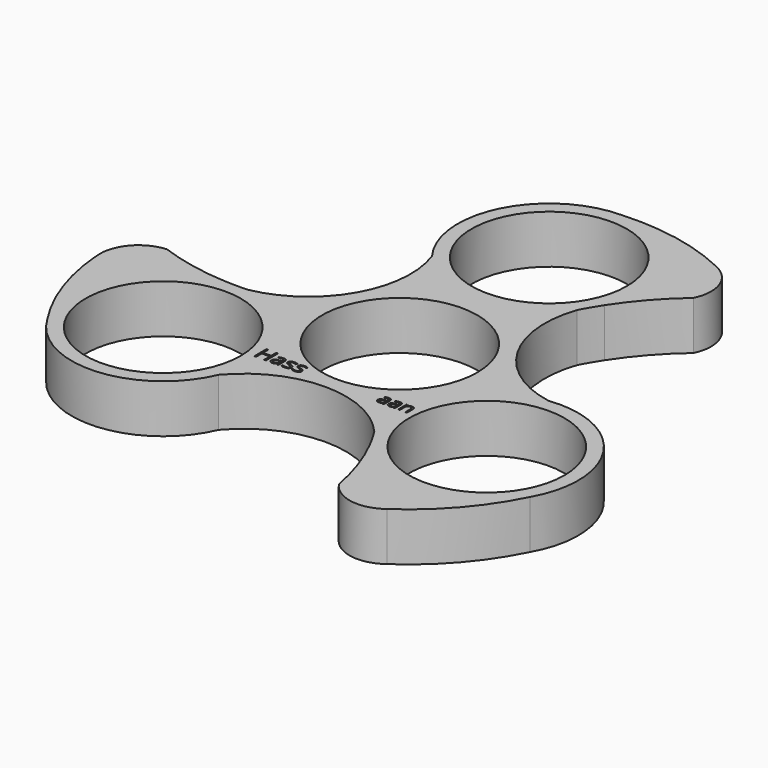
from build123d import *

# Parameters (mm, degrees)
F0_R         = 11.2
F1_DEPTH     = 7
F2_TEXT_SIZE = 3.0873436845
F3_DEPTH     = 13.4
F4_TEXT_SIZE = 2.8406800185
F5_DEPTH     = 9.9
F8_DEPTH     = 25


# Not quite as in the source:
# - Text() gives the source's letters only with a copy of the font that has no kerning and outlines rounded to 1/6400 em; it was checked with that copy


with BuildPart() as f1:
    # F0 (on Top) → F1 (new body)
    with BuildSketch(Plane.XY):
        with BuildLine():
            ThreePointArc((21.7602352684, -0.3790794713), (11.6629101979, 6.6669216362), (10.4657940357, 18.9212685418))
            ThreePointArc((10.4657940357, 18.9212685418), (11.2692033032, 20.371870284), (12.1401373601, 21.7829640918))
            ThreePointArc((12.1401373601, 21.7829640918), (17.0059122311, 27.7261145683), (23.0465047061, 32.4703790247))
            ThreePointArc((23.0465047061, 32.4703790247), (12.2370493927, 38.5690257647), (-0.0710858988, 40.165152914))
            ThreePointArc((-0.0710858988, 40.165152914), (-11.8253179711, 32.8306537694), (-10.551825182, 19.0344562705))
            ThreePointArc((-10.551825182, 19.0344562705), (-11.605178601, 6.7669156953), (-21.6191962469, -0.3969907652))
            ThreePointArc((-21.6191962469, -0.3969907652), (-23.2771588402, -0.426518801), (-24.9346689532, -0.3778146866))
            ThreePointArc((-24.9346689532, -0.3778146866), (-32.5144756799, 0.8644947226), (-39.643425459, 3.7236690316))
            ThreePointArc((-39.643425459, 3.7236690316), (-39.5202808078, -8.6869172409), (-34.748499821, -20.1441386512))
            ThreePointArc((-34.748499821, -20.1441386512), (-22.5195212016, -26.6563526555), (-11.2084100865, -18.6553767991))
            ThreePointArc((-11.2084100865, -18.6553767991), (-0.0577315969, -13.4338373316), (11.1534022111, -18.5242777766))
            ThreePointArc((11.1534022111, -18.5242777766), (12.0079555369, -19.945351483), (12.7945315932, -21.4051494051))
            ThreePointArc((12.7945315932, -21.4051494051), (15.5085634488, -28.5906092908), (16.5969207529, -36.1940480563))
            ThreePointArc((16.5969207529, -36.1940480563), (27.2832314151, -29.8821085238), (34.8195857199, -20.0210142628))
            ThreePointArc((34.8195857199, -20.0210142628), (34.3448391727, -6.1743011139), (21.7602352684, -0.3790794713))
        make_face()
        with Locations((-23.352673207, -13.4826721624)):
            Circle(F0_R, mode=Mode.SUBTRACT)
        Circle(F0_R, mode=Mode.SUBTRACT)
        with Locations((23.352673207, -13.4826721624)):
            Circle(F0_R, mode=Mode.SUBTRACT)
        with Locations((0, 26.9653443247)):
            Circle(F0_R, mode=Mode.SUBTRACT)
    extrude(amount=F1_DEPTH)

    # F2 (on face) → F3 (cut)
    with BuildSketch(Plane.XY.offset(7)):
        with Locations((-11.2112455724, -12.6004500012)):
            Text('Hass', F2_TEXT_SIZE, font='Open Sans', text_align=(TextAlign.LEFT, TextAlign.BOTTOM))
    extrude(amount=-F3_DEPTH, mode=Mode.SUBTRACT)

    # F4 (on face) → F5 (cut)
    with BuildSketch(Plane.XY.offset(7)):
        with Locations((6.4620403573, -12.6233948395)):
            Text('aan', F4_TEXT_SIZE, font='Open Sans', text_align=(TextAlign.LEFT, TextAlign.BOTTOM))
    extrude(amount=-F5_DEPTH, mode=Mode.SUBTRACT)

    # F7 (on face) → F8 (cut)
    with BuildSketch(Plane.XY.offset(7)):
        with BuildLine():
            ThreePointArc((-40.0765575469, -4.6404949389), (-38.8078254704, -0.355440868), (-34.801337868, 1.6243132995))
            ThreePointArc((-34.801337868, 1.6243132995), (-44.0770225904, 4.0814343372), (-40.0765575469, -4.6404949389))
        make_face()
        with BuildLine():
            ThreePointArc((24.0570652767, -32.3870694623), (19.7117335565, -33.430842289), (15.9939723529, -30.9509993291))
            ThreePointArc((15.9939723529, -30.9509993291), (18.5038854753, -40.212538455), (24.0570652767, -32.3870694623))
        make_face()
        with BuildLine():
            ThreePointArc((16.0194922702, 37.0275644013), (19.096091914, 33.786283157), (18.8073655151, 29.3266860296))
            ThreePointArc((18.8073655151, 29.3266860296), (25.5731371151, 36.1311041178), (16.0194922702, 37.0275644013))
        make_face()
    extrude(amount=-F8_DEPTH, mode=Mode.SUBTRACT)


solid = f1.part
